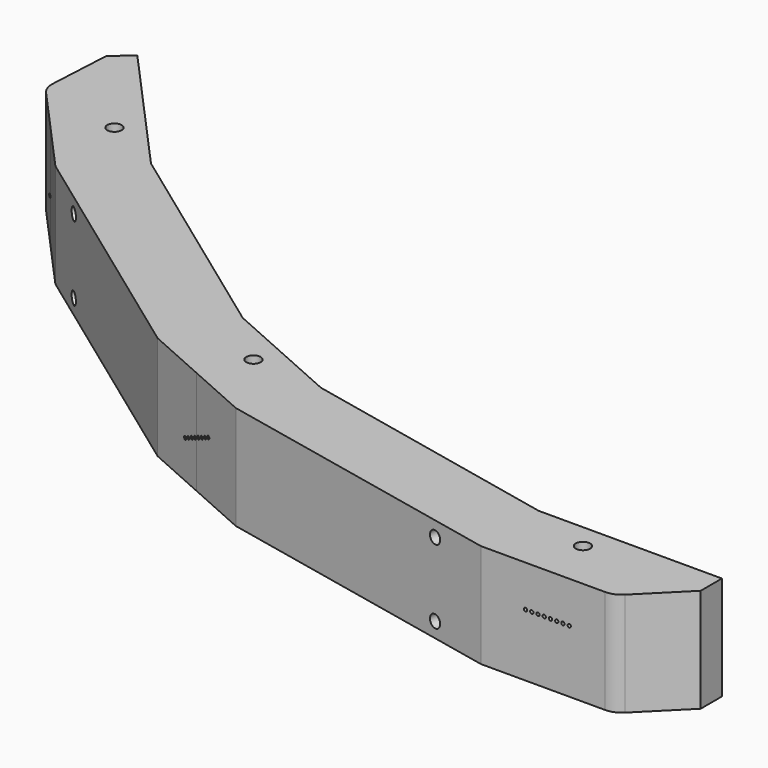
from build123d import *

# Parameters (mm, degrees)
F1_DEPTH        = 25
F2_W            = 13
F2_H            = 13
F3_DEPTH        = 10
F3_TAPER        = 3
F4_W            = 13
F4_H            = 13
F5_DEPTH        = 10
F5_TAPER        = 3
F7_D            = 0.8
F7_CSINK_D      = 0.866
F7_CSINK_ANGLE  = 60
F9_D            = 0.8
F9_CSINK_D      = 0.866
F9_CSINK_ANGLE  = 60
F10_W           = 13
F10_H           = 13
F11_DEPTH       = 10
F11_TAPER       = 3
F13_D           = 0.8
F13_CSINK_D     = 0.866
F13_CSINK_ANGLE = 60
F15_D           = 3.4544
F15_DEPTH       = 14.38125
F15_TIP         = 1.0378064612
F17_D           = 4.2
F17_DEPTH       = 10
F17_TIP         = 1.2618073
F18_R           = 0.3
F19_R           = 0.3
F20_R           = 0.3
F22_D           = 4.2
F22_DEPTH       = 10
F22_TIP         = 1.2618073
F24_D           = 4.2
F24_DEPTH       = 10
F24_TIP         = 1.2618073
F26_D           = 3.02
F28_D           = 3.02


# Not quite as in the source:
# - a feature names something its author has since deleted; it is built from what else it names


with BuildPart() as f1:
    # F0 (on Top) → F1 (new body)
    with BuildSketch(Plane.XY):
        with BuildLine():
            Line((-195.1064812103, -156.9314377097), (-185.7862063693, -167.2826515897))
            Line((-185.7862063693, -167.2826515897), (-175.0801166676, -179.1729687974))
            Line((-175.0801166676, -179.1729687974), (-116.3008880912, -221.8785781214))
            Line((-116.3008880912, -221.8785781214), (-101.6841607689, -228.3863644107))
            Line((-101.6841607689, -228.3863644107), (-87.0674334467, -234.8941506999))
            Line((-87.0674334467, -234.8941506999), (-16, -250))
            Line((-16, -250), (0, -250))
            Line((0, -250), (13.9289321881, -250))
            ThreePointArc((13.9289321881, -250), (15.84234935, -249.6193976626), (17.4644660941, -248.5355339059))
            Line((17.4644660941, -248.5355339059), (27.610408524, -238.389591476))
            Line((27.610408524, -238.389591476), (27.610408524, -232))
            Line((27.610408524, -232), (-0.4985836237, -232))
            Line((-0.4985836237, -232), (-16.4985836237, -232))
            Line((-16.4985836237, -232), (-79.7461738713, -218.4503324623))
            Line((-79.7461738713, -218.4503324623), (-94.3629011936, -211.9425461731))
            Line((-94.3629011936, -211.9425461731), (-108.9796285159, -205.4347598839))
            Line((-108.9796285159, -205.4347598839), (-161.703509809, -167.1286178829))
            Line((-161.703509809, -167.1286178829), (-172.4095995108, -155.2383006753))
            Line((-172.4095995108, -155.2383006753), (-191.2181864707, -134.3492486113))
            Line((-191.2181864707, -134.3492486113), (-195.596058473, -138.2911022675))
            Line((-195.596058473, -138.2911022675), (-196.3839047567, -153.3241048967))
            ThreePointArc((-196.3839047567, -153.3241048967), (-196.1039645384, -155.2548189741), (-195.1064812103, -156.9314377097))
        make_face()
    extrude(amount=-F1_DEPTH)

    # F2 (on face) → F3 (cut)
    with BuildSketch(Plane(origin=(-94.3629011936, -211.9425461731, 0), x_dir=(-0.9135454576, 0.4067366431, 0), z_dir=(0.4067366431, 0.9135454576, 0))):
        with Locations((0, -12.5)):
            Rectangle(F2_W, F2_H)
    extrude(amount=-F3_DEPTH, taper=F3_TAPER, mode=Mode.SUBTRACT)

    # F4 (on face) → F5 (cut)
    with BuildSketch(Plane(origin=(-172.4095995108, -155.2383006753, 0), x_dir=(-0.6691306064, 0.7431448255, 0), z_dir=(0.7431448255, 0.6691306064, 0))):
        with Locations((0, -12.5)):
            Rectangle(F4_W, F4_H)
    extrude(amount=-F5_DEPTH, taper=F5_TAPER, mode=Mode.SUBTRACT)

    # F7 (through all)
    with Locations(Plane(origin=(-179.8410477655, -161.9296067388, 0), x_dir=(-0.6691306064, 0.7431448255, 0), z_dir=(0.7431448255, 0.6691306064, 0))):
        with Locations((4.7581158819, -16.9134139554), (3.3986542014, -16.2794865628), (2.0391925208, -15.6455591702), (0.6797308403, -15.0116317776), (-0.6797308403, -14.377704385), (-2.0391925208, -13.7437769924), (-3.3986542014, -13.1098495998), (-4.7581158819, -12.4759222072)):
            CounterSinkHole(F7_D / 2, F7_CSINK_D / 2, counter_sink_angle=F7_CSINK_ANGLE)

    # F9 (through all)
    with Locations(Plane(origin=(-98.4302676243, -221.0780007495, 0), x_dir=(-0.9135454576, 0.4067366431, 0), z_dir=(0.4067366431, 0.9135454576, 0))):
        with Locations((4.7581158819, -15.9134139554), (3.3986542014, -15.2794865628), (2.0391925208, -14.6455591702), (0.6797308403, -14.0116317776), (-0.6797308403, -13.377704385), (-2.0391925208, -12.7437769924), (-3.3986542014, -12.1098495998), (-4.7581158819, -11.4759222072)):
            CounterSinkHole(F9_D / 2, F9_CSINK_D / 2, counter_sink_angle=F9_CSINK_ANGLE)

    # F10 (on face) → F11 (cut)
    with BuildSketch(Plane(origin=(0, -232, 0), x_dir=(-1, 0, 0), z_dir=(0, 1, 0))):
        with Locations((0, -12.5)):
            Rectangle(F10_W, F10_H)
    extrude(amount=-F11_DEPTH, taper=F11_TAPER, mode=Mode.SUBTRACT)

    # F13 (through all)
    with Locations(Plane(origin=(0, -242, 0), x_dir=(-1, 0, 0), z_dir=(0, 1, 0))):
        with Locations((5.25, -9.9759222072), (3.75, -9.9759222072), (2.25, -9.9759222072), (0.75, -9.9759222072), (-0.75, -9.9759222072), (-2.25, -9.9759222072), (-3.75, -9.9759222072), (-5.25, -9.9759222072)):
            CounterSinkHole(F13_D / 2, F13_CSINK_D / 2, counter_sink_angle=F13_CSINK_ANGLE)

    # F15
    with Locations(Plane.XY):
        with Locations((-176.1755610332, -160.0226359772), (-96.803321052, -217.4238189189), (-1.0355339059, -238)):
            Hole(F15_D / 2, depth=F15_DEPTH)
            with Locations((0, 0, -(F15_DEPTH + F15_TIP / 2))):  # 118° drill point
                Cone(0, F15_D / 2, F15_TIP, mode=Mode.SUBTRACT)

    # F17
    with Locations(Plane(origin=(0, -232, 0), x_dir=(-1, 0, 0), z_dir=(0, 1, 0))):
        with Locations((13.2492918119, -4.3), (13.2492918119, -20.7), (-18.560408524, -4.3), (-18.560408524, -20.7)):
            Hole(F17_D / 2, depth=F17_DEPTH)
            with Locations((0, 0, -(F17_DEPTH + F17_TIP / 2))):  # 118° drill point
                Cone(0, F17_D / 2, F17_TIP, mode=Mode.SUBTRACT)

    # F18
    f18_edges = [f1.edges().sort_by_distance(p)[0] for p in [
        (-5.975922, -242, -12.5),
        (0, -242, -6.524078),
        (5.975922, -242, -12.5),
        (0, -242, -18.475922),
        (-6.237961, -237, -6.262039),
        (6.237961, -237, -6.262039),
        (6.237961, -237, -18.737961),
    ]]
    fillet(f18_edges, radius=F18_R)

    # F19
    f19_edges = [f1.edges().sort_by_distance(p)[0] for p in [
        (-98.430268, -221.078001, -6.524078),
        (-92.970991, -223.508627, -12.5),
        (-90.697923, -219.047481, -6.262039),
        (-90.697923, -219.047481, -18.737961),
        (-98.430268, -221.078001, -18.475922),
        (-103.889544, -218.647374, -12.5),
        (-102.095245, -213.973066, -6.262039),
        (-102.095245, -213.973066, -18.737961),
    ]]
    fillet(f19_edges, radius=F19_R)

    # F20
    f20_edges = [f1.edges().sort_by_distance(p)[0] for p in [
        (-179.841048, -161.929607, -18.475922),
        (-179.841048, -161.929607, -6.524078),
        (-175.842375, -166.370582, -12.5),
        (-171.951313, -163.219662, -6.262039),
        (-171.951313, -163.219662, -18.737961),
        (-183.83972, -157.488631, -12.5),
        (-180.299334, -153.948245, -6.262039),
        (-180.299334, -153.948245, -18.737961),
    ]]
    fillet(f20_edges, radius=F20_R)

    # F22
    with Locations(Plane(origin=(-94.3629011936, -211.9425461731, 0), x_dir=(-0.9135454576, 0.4067366431, 0), z_dir=(0.4067366431, 0.9135454576, 0))):
        with Locations((-13, -4.3), (-13, -20.7), (13, -4.3), (13, -20.7)):
            Hole(F22_D / 2, depth=F22_DEPTH)
            with Locations((0, 0, -(F22_DEPTH + F22_TIP / 2))):  # 118° drill point
                Cone(0, F22_D / 2, F22_TIP, mode=Mode.SUBTRACT)

    # F24
    with Locations(Plane(origin=(-172.4095995108, -155.2383006753, 0), x_dir=(-0.6691306064, 0.7431448255, 0), z_dir=(0.7431448255, 0.6691306064, 0))):
        with Locations((-13, -4.3), (-13, -20.7), (19.0589921478, -4.3), (19.0589921478, -20.7)):
            Hole(F24_D / 2, depth=F24_DEPTH)
            with Locations((0, 0, -(F24_DEPTH + F24_TIP / 2))):  # 118° drill point
                Cone(0, F24_D / 2, F24_TIP, mode=Mode.SUBTRACT)

    # F26 (through all)
    with Locations(Plane(origin=(-48.2448517048, -225.1989285856, 0), x_dir=(-0.9778131425, 0.2094790164, 0), z_dir=(0.2094790164, 0.9778131425, 0))):
        with Locations((-23.1390529194, -3.6051168097), (-23.1390529194, -21.3948831903)):
            Hole(F26_D / 2)

    # F28 (through all)
    with Locations(Plane(origin=(-135.3415691624, -186.2816888834, 0), x_dir=(-0.8090169944, 0.5877852523, 0), z_dir=(0.5877852523, 0.8090169944, 0))):
        with Locations((23.2485540845, -3.5816147789), (23.2485540845, -21.4183852211)):
            Hole(F28_D / 2)


solid = f1.part
